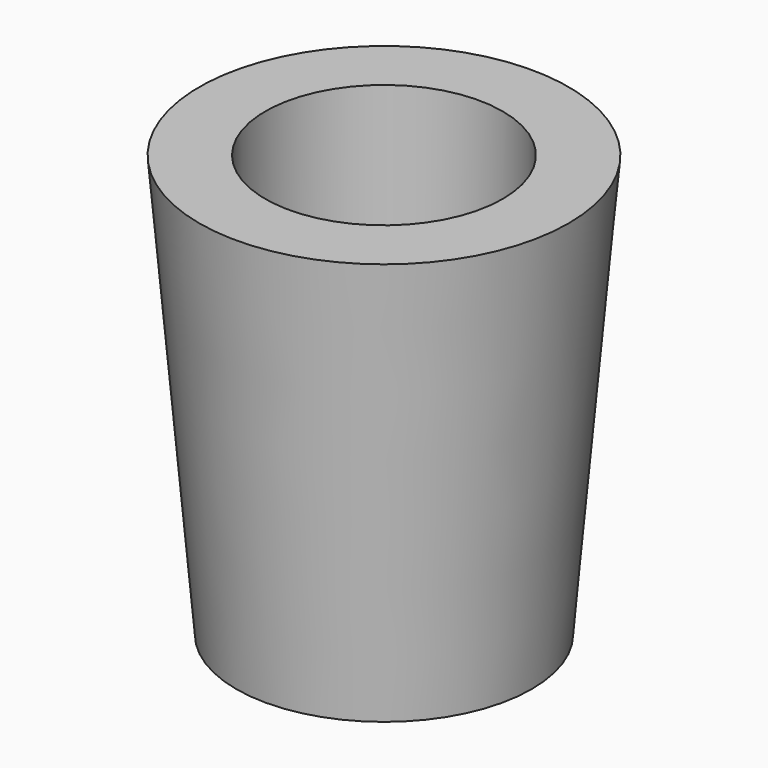
from build123d import *

# Parameters (mm, degrees)
F0_R     = 35
F0_R_2   = 22.5
F1_DEPTH = 80
F2_SIZE2 = 6.999083
F2_SIZE  = 79.99999


# Not quite as in the source:
# - a fillet or chamfer is up to 0.001 mm smaller than in the source, because OpenCascade refuses the exact size


with BuildPart() as f1:
    # F0 (on Top) → F1 (new body)
    with BuildSketch(Plane.XY):
        Circle(F0_R)
        Circle(F0_R_2, mode=Mode.SUBTRACT)
    extrude(amount=F1_DEPTH)

    # F2 (size 80 and 6.9990930821 in the source; OpenCascade refuses exactly that, so slightly less here)
    f2_edges = [f1.edges().sort_by_distance(p)[0] for p in [
        (-35, 0, 0),
    ]]
    f2_side = f1.faces().sort_by_distance((-35, 0, 40))[0]
    chamfer(f2_edges, length=F2_SIZE, length2=F2_SIZE2, reference=f2_side)


solid = f1.part
